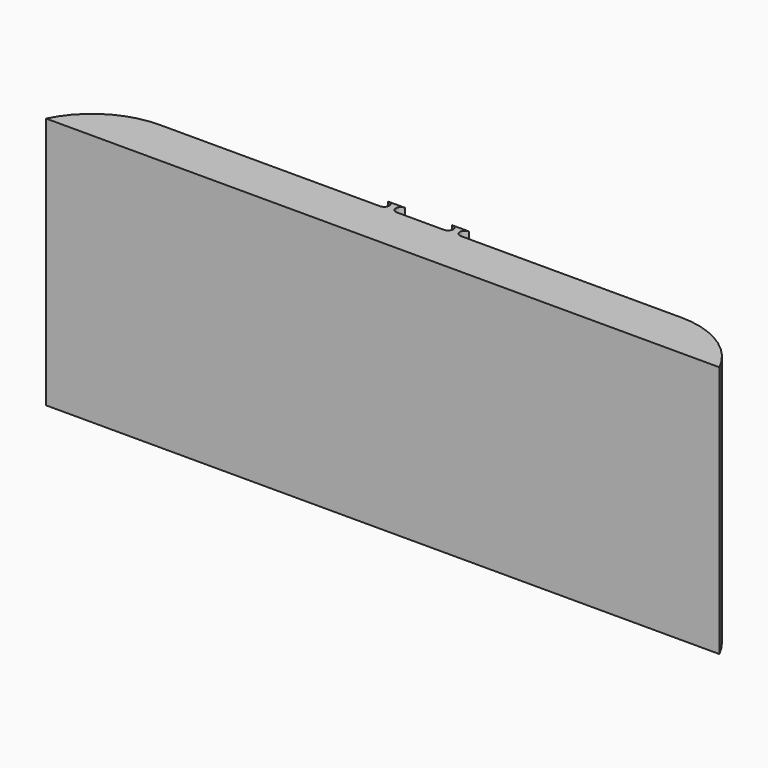
from build123d import *

# Parameters (mm, degrees)
F0_R     = 5.25
F1_DEPTH = 75
F4_DEPTH = 2


# Not quite as in the source:
# - a feature names something its author has since deleted; it is built from what else it names


with BuildPart() as f1:
    # F0 (on Top) → F1 (new body)
    with BuildSketch(Plane.XY):
        with BuildLine():
            Line((-100, 0), (-13.8524602948, 0))
            Line((-13.8524602948, 0), (12.09906023, 0))
            Line((12.09906023, 0), (100, 0))
            ThreePointArc((100, 0), (90.75, 10.2142857143), (77.5, 14))
            Line((77.5, 14), (32.5911540906, 14))
            Line((32.5911540906, 14), (26.9999997473, 14))
            Line((26.9999997473, 14), (11.9999997473, 14))
            Line((11.9999997473, 14), (7, 14))
            Line((7, 14), (-7, 14))
            Line((-7, 14), (-11.9999997473, 14))
            Line((-11.9999997473, 14), (-77.5, 14))
            ThreePointArc((-77.5, 14), (-90.75, 10.2142857143), (-100, 0))
        make_face()
        with Locations((0, 7.25)):
            Circle(F0_R, mode=Mode.SUBTRACT)
        with Locations((30.1251118069, 7.25)):
            Circle(F0_R, mode=Mode.SUBTRACT)
        with Locations((30.1251118069, 7.25)):
            Circle(F0_R)
        with BuildLine():
            ThreePointArc((-11.9999997473, 17), (-10.4999997473, 15.5), (-11.9999997473, 14))
            Line((-11.9999997473, 14), (-7, 14))
            ThreePointArc((-7, 14), (-8.5, 15.5000001263), (-6.9999997473, 17))
            Line((-6.9999997473, 17), (-11.9999997473, 17))
        make_face()
        with BuildLine():
            ThreePointArc((6.9999998542, 17), (8.5, 15.5000000729), (7, 14))
            Line((7, 14), (11.9999997473, 14))
            ThreePointArc((11.9999997473, 14), (10.4999997473, 15.5), (11.9999997473, 17))
            Line((11.9999997473, 17), (6.9999998542, 17))
        make_face()
        with Locations((0, 7.25)):
            Circle(F0_R)
    extrude(amount=F1_DEPTH)

    # F0 (on Top) → F4 (join)
    with BuildSketch(Plane.XY):
        with BuildLine():
            ThreePointArc((11.9999997473, 17), (10.4999997473, 15.5), (11.9999997473, 14))
            Line((11.9999997473, 14), (11.9999997473, 17))
        make_face()
        with BuildLine():
            Line((6.9999998542, 17), (7, 14))
            ThreePointArc((7, 14), (8.5, 15.5000000729), (6.9999998542, 17))
        make_face()
        with BuildLine():
            ThreePointArc((-6.9999997473, 17), (-8.5, 15.5000001263), (-7, 14))
            Line((-7, 14), (-6.9999997473, 17))
        make_face()
        with BuildLine():
            Line((-11.9999997473, 17), (-11.9999997473, 14))
            ThreePointArc((-11.9999997473, 14), (-10.4999997473, 15.5), (-11.9999997473, 17))
        make_face()
        with BuildLine():
            ThreePointArc((-11.9999997473, 17), (-10.4999997473, 15.5), (-11.9999997473, 14))
            Line((-11.9999997473, 14), (-7, 14))
            ThreePointArc((-7, 14), (-8.5, 15.5000001263), (-6.9999997473, 17))
            Line((-6.9999997473, 17), (-11.9999997473, 17))
        make_face()
        with BuildLine():
            ThreePointArc((6.9999998542, 17), (8.5, 15.5000000729), (7, 14))
            Line((7, 14), (11.9999997473, 14))
            ThreePointArc((11.9999997473, 14), (10.4999997473, 15.5), (11.9999997473, 17))
            Line((11.9999997473, 17), (6.9999998542, 17))
        make_face()
    extrude(amount=F4_DEPTH)

    # F5: sweep along a path in F3
    with BuildLine(Plane.YZ.offset(30.1251118069)) as f5_path:
        Line((8, 0), (8, 23))
        Line((8, 23), (14, 23))
    # F0 (on Top) → F5 (sweep, cut)
    with BuildSketch(Plane.XY):
        with Locations((30.1251118069, 7.25)):
            Circle(F0_R)
    sweep(path=f5_path.line, transition=Transition.RIGHT, mode=Mode.SUBTRACT)

    # F7: sweep along a path in F6
    with BuildLine(Plane.YZ) as f7_path:
        Line((23.7799418298, 13.885), (9.2960403562, 13.885))
        Line((9.2960403562, 13.885), (9.2960403562, 0))
    # F0 (on Top) → F7 (sweep, cut)
    with BuildSketch(Plane.XY):
        with Locations((0, 7.25)):
            Circle(F0_R)
    sweep(path=f7_path.line, transition=Transition.RIGHT, mode=Mode.SUBTRACT)


solid = f1.part
